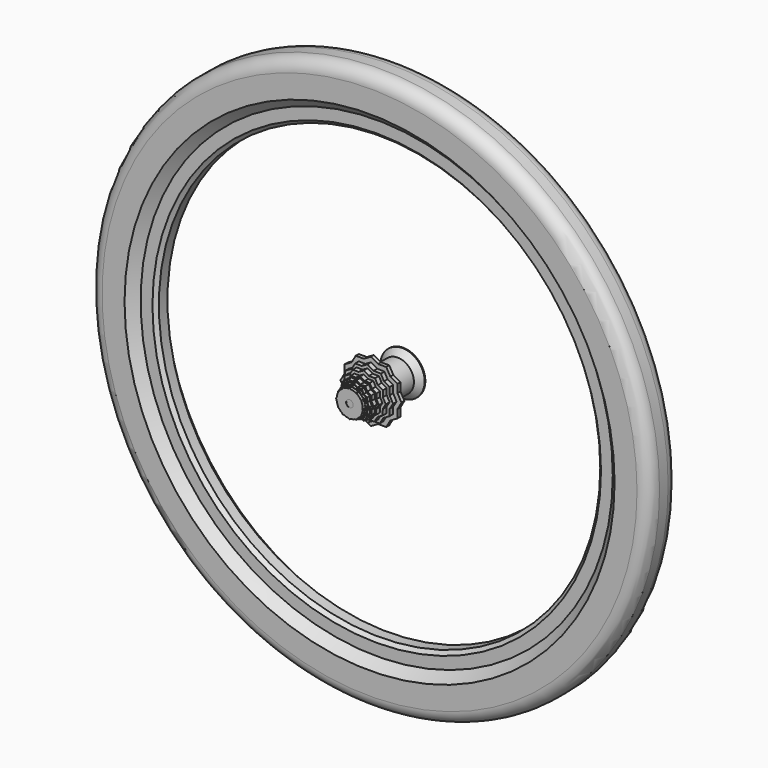
from build123d import *

# Parameters (mm, degrees)
F0_R        = 330.2
F0_R_2      = 313.4398178368
F1_DEPTH    = 12.7
F2_SIZE     = 5.08
F3_R        = 23.0340287743
F4_DEPTH    = 12.7
F5_R        = 31.4850250761
F6_DEPTH    = 21.59
F7_R        = 31.4849467141
F8_DEPTH    = 4.826
F9_S5_R     = 23.0340287743
F9_T6_DEPTH = 47
F10_R       = 18.571291292
F11_DEPTH   = 43.18
F12_R       = 31.4849467141
F13_DEPTH   = 5.334
F15_DEPTH   = 6.35
F17_DEPTH   = 6.858
F19_DEPTH   = 6.35
F21_DEPTH   = 6.35
F23_DEPTH   = 4.572
F25_DEPTH   = 3.302
F27_DEPTH   = 3.8862
F28_R       = 5
F29_DEPTH   = 118.11
F30_R       = 397.6407054021
F30_R_2     = 330.2
F31_DEPTH   = 25.4
F33_R       = 17.78


# Not quite as in the source:
# - a fillet or chamfer that OpenCascade refuses, or shapes differently, is made with other operations: its cross-section is extruded or revolved along the edge and cut away or added


with BuildPart() as f1:
    # F0 (on Front) → F1 (new body, symmetric)
    with BuildSketch(Plane.XZ):
        Circle(F0_R)
        Circle(F0_R_2, mode=Mode.SUBTRACT)
    extrude(amount=F1_DEPTH, both=True)

    # F2
    f2_edges = [f1.edges().sort_by_distance(p)[0] for p in [
        (-313.439818, -12.7, 0),
        (-313.439818, 12.7, 0),
    ]]
    chamfer(f2_edges, length=F2_SIZE)

    # F30 (on Front) → F31 (join, symmetric)
    with BuildSketch(Plane.XZ):
        Circle(F30_R)
        Circle(F30_R_2, mode=Mode.SUBTRACT)
    extrude(amount=F31_DEPTH, both=True)

    # F32: chamfer of 17.78 on 1 edges, made by hand


with BuildPart() as f4:
    # F3 (on Front) → F4 (new body, symmetric)
    with BuildSketch(Plane.XZ):
        Circle(F3_R)
    extrude(amount=F4_DEPTH, both=True)

    # F5 (on face) → F6 (join)
    with BuildSketch(Plane(origin=(0, 12.7, 0), x_dir=(-1, 0, 0), z_dir=(0, 1, 0))):
        Circle(F5_R)
    extrude(amount=F6_DEPTH)

    # F7 (on face) → F8 (join)
    with BuildSketch(Plane.XZ.offset(12.7)):
        Circle(F7_R)
    extrude(amount=F8_DEPTH)

    # F9: chamfer of 20.32 on 1 edges, made by hand


with BuildPart() as f9_tool2:
    # F9_s3 → F9_t4 (revolve)
    with BuildSketch(Plane.XY):
        Polygon((-11.1650250761, 12.7), (-31.4850250761, 33.02), (-31.4850250761, 12.7), align=None)
    revolve(axis=Axis((0, 12.7, 0), (0, 1, 0)))

    # F9_s5 → F9_t6 (cut, symmetric)
    with BuildSketch(Plane.XZ.offset(-22.9)):
        Circle(F9_S5_R)
    extrude(amount=F9_T6_DEPTH, both=True, mode=Mode.SUBTRACT)


with BuildPart() as f4_1:
    add(f4.part)

    # F9_t1: cut F9_tool2
    add(f9_tool2.part, mode=Mode.SUBTRACT)

    # F10 (on face) → F11 (join)
    with BuildSketch(Plane.XZ.offset(17.526)):
        Circle(F10_R)
    extrude(amount=F11_DEPTH)

    # F28 (on face) → F29 (cut)
    with BuildSketch(Plane.XZ.offset(60.706)):
        Circle(F28_R)
    extrude(amount=-F29_DEPTH, mode=Mode.SUBTRACT)


with BuildPart() as f13:
    # F12 (on face) → F13 (new body)
    with BuildSketch(Plane.XZ.offset(17.526)):
        Polygon((37.5246405602, -10.0546971344), (37.5246405602, 10.0546971344), (27.4699434258, 27.4699434258), (10.0546971344, 37.5246405602), (-10.0546971344, 37.5246405602), (-27.4699434258, 27.4699434258), (-37.5246405602, 10.0546971344), (-37.5246405602, -10.0546971344), (-27.4699434258, -27.4699434258), (-10.0546971344, -37.5246405602), (10.0546971344, -37.5246405602), (27.4699434258, -27.4699434258), align=None)
        Circle(F12_R, mode=Mode.SUBTRACT)
        Polygon((10.0546971344, 37.5246405602), (27.4699434258, 27.4699434258), (21.6648613286, 37.5246405602), align=None)
        Polygon((-27.4699434258, 27.4699434258), (-10.0546971344, 37.5246405602), (-21.6648613286, 37.5246405602), align=None)
        Polygon((-10.0546971344, 37.5246405602), (10.0546971344, 37.5246405602), (0, 43.3297226573), align=None)
        Polygon((-37.5246405602, 10.0546971344), (-27.4699434258, 27.4699434258), (-37.5246405602, 21.6648613286), align=None)
        Polygon((-37.5246405602, -10.0546971344), (-37.5246405602, 10.0546971344), (-43.3297226573, 0), align=None)
        Polygon((-37.5246405602, -21.6648613286), (-27.4699434258, -27.4699434258), (-37.5246405602, -10.0546971344), align=None)
        Polygon((-21.6648613286, -37.5246405602), (-10.0546971344, -37.5246405602), (-27.4699434258, -27.4699434258), align=None)
        Polygon((0, -43.3297226573), (10.0546971344, -37.5246405602), (-10.0546971344, -37.5246405602), align=None)
        Polygon((21.6648613286, -37.5246405602), (27.4699434258, -27.4699434258), (10.0546971344, -37.5246405602), align=None)
        Polygon((37.5246405602, -21.6648613286), (37.5246405602, -10.0546971344), (27.4699434258, -27.4699434258), align=None)
        Polygon((43.3297226573, 0), (37.5246405602, 10.0546971344), (37.5246405602, -10.0546971344), align=None)
        Polygon((37.5246405602, 10.0546971344), (37.5246405602, 21.6648613286), (27.4699434258, 27.4699434258), align=None)
    extrude(amount=F13_DEPTH)


with BuildPart() as f15:
    # F14 (on face) → F15 (new body)
    with BuildSketch(Plane.XZ.offset(22.86)):
        Polygon((31.4849467141, 7.9340602855), (31.4849467141, 18.1778424608), (23.487088156, 22.7954082522), align=None)
        Polygon((36.3394488072, -1.0864099174), (31.4849467141, 7.9340602855), (31.4849467141, -8.9427108779), align=None)
        Polygon((31.4849467141, -8.9427108779), (31.4849467141, 7.9340602855), (23.487088156, 22.7954082522), (8.8713755946, 31.2337938339), (-7.9978585581, 31.7381191301), (-22.6135711195, 23.2997335484), (-31.4849467141, 8.9427108779), (-31.4849467141, -7.9340602855), (-23.487088156, -22.7954082522), (-8.8713755946, -31.2337938339), (7.9978585581, -31.7381191301), (22.6135711195, -23.2997335484), align=None)
        Polygon((8.8713755946, 31.2337938339), (23.487088156, 22.7954082522), (19.110582991, 30.9276808678), align=None)
        Polygon((31.4849467141, -18.1778424608), (31.4849467141, -8.9427108779), (22.6135711195, -23.2997335484), align=None)
        Polygon((-7.9978585581, 31.7381191301), (8.8713755946, 31.2337938339), (0, 36.3556849216), align=None)
        Polygon((17.2288658162, -32.0140907852), (22.6135711195, -23.2997335484), (7.9978585581, -31.7381191301), align=None)
        Polygon((-22.6135711195, 23.2997335484), (-7.9978585581, 31.7381191301), (-17.2288658162, 32.0140907852), align=None)
        Polygon((0, -36.3556849216), (7.9978585581, -31.7381191301), (-8.8713755946, -31.2337938339), align=None)
        Polygon((-31.4849467141, 8.9427108779), (-22.6135711195, 23.2997335484), (-31.4849467141, 18.1778424608), align=None)
        Polygon((-19.110582991, -30.9276808678), (-8.8713755946, -31.2337938339), (-23.487088156, -22.7954082522), align=None)
        Polygon((-31.4849467141, -7.9340602855), (-31.4849467141, 8.9427108779), (-36.3394488072, 1.0864099174), align=None)
        Polygon((-31.4849467141, -18.1778424608), (-23.487088156, -22.7954082522), (-31.4849467141, -7.9340602855), align=None)
    extrude(amount=F15_DEPTH)


with BuildPart() as f17:
    # F16 (on face) → F17 (new body)
    with BuildSketch(Plane.XZ.offset(29.21)):
        Polygon((7.6229792377, 27.1815358473), (0.1521180714, 31.5430119156), (-7.0145946523, 27.451262981), align=None)
        Polygon((16.272305085, 27.0221543892), (7.6229792377, 27.1815358473), (20.2661937814, 19.8004486566), align=None)
        Polygon((20.2661937814, 19.8004486566), (7.6229792377, 27.1815358473), (-7.0145946523, 27.451262981), (-19.7284109388, 20.1924615961), (-27.2807884337, 7.6508143244), (-27.3513901765, -6.9890742513), (-20.2661937814, -19.8004486566), (-7.6229792377, -27.1815358473), (7.0145946523, -27.451262981), (19.7284109388, -20.1924615961), (27.2807884337, -7.6508143244), (27.3513901765, 6.9890742513), align=None)
        Polygon((-19.7284109388, 20.1924615961), (-7.0145946523, 27.451262981), (-15.2657196236, 27.6033067763), align=None)
        Polygon((27.3931086665, 15.6397678436), (20.2661937814, 19.8004486566), (27.3513901765, 6.9890742513), align=None)
        Polygon((-27.2807884337, 7.6508143244), (-19.7284109388, 20.1924615961), (-27.2409905951, 15.903244072), align=None)
        Polygon((31.5380247085, -0.5811523871), (27.3513901765, 6.9890742513), (27.2807884337, -7.6508143244), align=None)
        Polygon((-27.3513901765, -6.9890742513), (-27.2807884337, 7.6508143244), (-31.5380247085, 0.5811523871), align=None)
        Polygon((27.2409905951, -15.903244072), (27.2807884337, -7.6508143244), (19.7284109388, -20.1924615961), align=None)
        Polygon((-20.2661937814, -19.8004486566), (-27.3513901765, -6.9890742513), (-27.3931086665, -15.6397678436), align=None)
        Polygon((15.2657196236, -27.6033067763), (19.7284109388, -20.1924615961), (7.0145946523, -27.451262981), align=None)
        Polygon((-7.6229792377, -27.1815358473), (-20.2661937814, -19.8004486566), (-16.272305085, -27.0221543892), align=None)
        Polygon((-0.1521180714, -31.5430119156), (7.0145946523, -27.451262981), (-7.6229792377, -27.1815358473), align=None)
    extrude(amount=F17_DEPTH)


with BuildPart() as f19:
    # F18 (on face) → F19 (new body)
    with BuildSketch(Plane.XZ.offset(36.068)):
        Polygon((6.6182012985, 23.1333943168), (0.4520852324, 26.8332787451), (-5.8351667066, 23.3432078034), align=None)
        Polygon((13.8081566685, 23.0122584439), (6.6182012985, 23.1333943168), (17.2982276102, 16.7250065049), align=None)
        Polygon((17.2982276102, 16.7250065049), (6.6182012985, 23.1333943168), (-5.8351667066, 23.3432078034), (-16.7250065049, 17.2982276102), (-23.1333943168, 6.6182012985), (-23.3432078034, -5.8351667066), (-17.2982276102, -16.7250065049), (-6.6182012985, -23.1333943168), (5.8351667066, -23.3432078034), (16.7250065049, -17.2982276102), (23.1333943168, -6.6182012985), (23.3432078034, 5.8351667066), align=None)
        Polygon((-16.7250065049, 17.2982276102), (-5.8351667066, 23.3432078034), (-13.0251220766, 23.4643436763), align=None)
        Polygon((23.4643436763, 13.0251220766), (17.2982276102, 16.7250065049), (23.3432078034, 5.8351667066), align=None)
        Polygon((-23.1333943168, 6.6182012985), (-16.7250065049, 17.2982276102), (-23.0122584439, 13.8081566685), align=None)
        Polygon((26.8332787451, -0.4520852324), (23.3432078034, 5.8351667066), (23.1333943168, -6.6182012985), align=None)
        Polygon((-23.3432078034, -5.8351667066), (-23.1333943168, 6.6182012985), (-26.8332787451, 0.4520852324), align=None)
        Polygon((23.0122584439, -13.8081566685), (23.1333943168, -6.6182012985), (16.7250065049, -17.2982276102), align=None)
        Polygon((-17.2982276102, -16.7250065049), (-23.3432078034, -5.8351667066), (-23.4643436763, -13.0251220766), align=None)
        Polygon((13.0251220766, -23.4643436763), (16.7250065049, -17.2982276102), (5.8351667066, -23.3432078034), align=None)
        Polygon((-6.6182012985, -23.1333943168), (-17.2982276102, -16.7250065049), (-13.8081566685, -23.0122584439), align=None)
        Polygon((-0.4520852324, -26.8332787451), (5.8351667066, -23.3432078034), (-6.6182012985, -23.1333943168), align=None)
    extrude(amount=F19_DEPTH)


with BuildPart() as f21:
    # F20 (on face) → F21 (new body)
    with BuildSketch(Plane.XZ.offset(42.418)):
        Polygon((15.6329888137, 15.4468506512), (12.497079395, 21.0376595296), (5.795126247, 21.1209169034), align=None)
        Polygon((21.1858358601, 12.2442015171), (15.6329888137, 15.4468506512), (21.1888137131, 5.5417319036), align=None)
        Polygon((21.1888137131, 5.5417319036), (15.6329888137, 15.4468506512), (5.795126247, 21.1209169034), (-5.5608706655, 21.2619907753), (-15.393687466, 15.5791849997), (-21.1938594792, 5.8151401242), (-21.1888137131, -5.5417319036), (-15.6329888137, -15.4468506512), (-5.795126247, -21.1209169034), (5.5608706655, -21.2619907753), (15.393687466, -15.5791849997), (21.1938594792, -5.8151401242), align=None)
        Polygon((-5.5608706655, 21.2619907753), (5.795126247, 21.1209169034), (-0.0108716328, 24.4695728139), align=None)
        Polygon((24.4676872862, -0.3039584644), (21.1888137131, 5.5417319036), (21.1938594792, -5.8151401242), align=None)
        Polygon((-15.393687466, 15.5791849997), (-5.5608706655, 21.2619907753), (-11.9706078913, 21.3416179939), align=None)
        Polygon((21.196707493, -12.2253712967), (21.1938594792, -5.8151401242), (15.393687466, -15.5791849997), align=None)
        Polygon((-21.1938594792, 5.8151401242), (-15.393687466, 15.5791849997), (-21.196707493, 12.2253712967), align=None)
        Polygon((11.9706078913, -21.3416179939), (15.393687466, -15.5791849997), (5.5608706655, -21.2619907753), align=None)
        Polygon((-21.1888137131, -5.5417319036), (-21.1938594792, 5.8151401242), (-24.4676872862, 0.3039584644), align=None)
        Polygon((0.0108716328, -24.4695728139), (5.5608706655, -21.2619907753), (-5.795126247, -21.1209169034), align=None)
        Polygon((-15.6329888137, -15.4468506512), (-21.1888137131, -5.5417319036), (-21.1858358601, -12.2442015171), align=None)
        Polygon((-12.497079395, -21.0376595296), (-5.795126247, -21.1209169034), (-15.6329888137, -15.4468506512), align=None)
    extrude(amount=F21_DEPTH)


with BuildPart() as f23:
    # F22 (on face) → F23 (new body)
    with BuildSketch(Plane.XZ.offset(48.768)):
        Polygon((14.1206154101, 13.8263447779), (11.4125081967, 18.7722549839), (5.2812427209, 18.9111061399), align=None)
        Polygon((19.0084046936, 11.0146925297), (14.1206154101, 13.8263447779), (19.0181196913, 4.8818627101), align=None)
        Polygon((19.0181196913, 4.8818627101), (14.1206154101, 13.8263447779), (5.2812427209, 18.9111061399), (-4.9136581141, 19.1419840512), (-13.7368769704, 14.0292434299), (-19.0342735242, 5.3156392733), (-19.0181196913, -4.8818627101), (-14.1206154101, -13.8263447779), (-5.2812427209, -18.9111061399), (4.9136581141, -19.1419840512), (13.7368769704, -14.0292434299), (19.0342735242, -5.3156392733), align=None)
        Polygon((-4.9136581141, 19.1419840512), (5.2812427209, 18.9111061399), (-0.0348011988, 21.969107615), align=None)
        Polygon((21.9635038007, -0.4973945273), (19.0181196913, 4.8818627101), (19.0342735242, -5.3156392733), align=None)
        Polygon((-13.7368769704, 14.0292434299), (-4.9136581141, 19.1419840512), (-10.550995604, 19.2696495112), align=None)
        Polygon((19.0432058924, -10.9544150852), (19.0342735242, -5.3156392733), (13.7368769704, -14.0292434299), align=None)
        Polygon((-19.0342735242, 5.3156392733), (-13.7368769704, 14.0292434299), (-19.0432058924, 10.9544150852), align=None)
        Polygon((10.550995604, -19.2696495112), (13.7368769704, -14.0292434299), (4.9136581141, -19.1419840512), align=None)
        Polygon((-19.0181196913, -4.8818627101), (-19.0342735242, 5.3156392733), (-21.9635038007, 0.4973945273), align=None)
        Polygon((0.0348011988, -21.969107615), (4.9136581141, -19.1419840512), (-5.2812427209, -18.9111061399), align=None)
        Polygon((-14.1206154101, -13.8263447779), (-19.0181196913, -4.8818627101), (-19.0084046936, -11.0146925297), align=None)
        Polygon((-11.4125081967, -18.7722549839), (-5.2812427209, -18.9111061399), (-14.1206154101, -13.8263447779), align=None)
    extrude(amount=F23_DEPTH)


with BuildPart() as f25:
    # F24 (on face) → F25 (new body)
    with BuildSketch(Plane.XZ.offset(53.34)):
        Polygon((4.9557047364, 17.8605892728), (-0.0098370627, 20.7243044155), (-4.6617860124, 18.0355554854), align=None)
        Polygon((10.686899955, 17.7563244966), (4.9557047364, 17.8605892728), (13.2883562156, 13.0550028564), align=None)
        Polygon((13.2883562156, 13.0550028564), (4.9557047364, 17.8605892728), (-4.6617860124, 18.0355554854), (-12.9898716686, 13.2220608318), (-17.9501422279, 4.980552629), (-17.945576405, -4.638528441), (-13.2883562156, -13.0550028564), (-4.9557047364, -17.8605892728), (4.6617860124, -18.0355554854), (12.9898716686, -13.2220608318), (17.9501422279, -4.980552629), (17.945576405, 4.638528441), align=None)
        Polygon((-12.9898716686, 13.2220608318), (-4.6617860124, 18.0355554854), (-10.0339781144, 18.133289097), align=None)
        Polygon((17.9428555683, 10.370671354), (13.2883562156, 13.0550028564), (17.945576405, 4.638528441), align=None)
        Polygon((-17.9501422279, 4.980552629), (-12.9898716686, 13.2220608318), (-17.952692631, 10.3536330616), align=None)
        Polygon((20.7208780694, -0.3769646005), (17.945576405, 4.638528441), (17.9501422279, -4.980552629), align=None)
        Polygon((-17.945576405, -4.638528441), (-17.9501422279, 4.980552629), (-20.7208780694, 0.3769646005), align=None)
        Polygon((17.952692631, -10.3536330616), (17.9501422279, -4.980552629), (12.9898716686, -13.2220608318), align=None)
        Polygon((-13.2883562156, -13.0550028564), (-17.945576405, -4.638528441), (-17.9428555683, -10.370671354), align=None)
        Polygon((10.0339781144, -18.133289097), (12.9898716686, -13.2220608318), (4.6617860124, -18.0355554854), align=None)
        Polygon((-4.9557047364, -17.8605892728), (-13.2883562156, -13.0550028564), (-10.686899955, -17.7563244966), align=None)
        Polygon((0.0098370627, -20.7243044155), (4.6617860124, -18.0355554854), (-4.9557047364, -17.8605892728), align=None)
    extrude(amount=F25_DEPTH)


with BuildPart() as f27:
    # F26 (on face) → F27 (new body)
    with BuildSketch(Plane.XZ.offset(56.642)):
        Polygon((4.7735277821, 16.8202055695), (0.0513016488, 19.5631203379), (-4.3039365876, 17.0638273834), align=None)
        Polygon((10.2326060501, 16.6736943307), (4.7735277821, 16.8202055695), (12.625739706, 12.2592321128), align=None)
        Polygon((12.625739706, 12.2592321128), (4.7735277821, 16.8202055695), (-4.3039365876, 17.0638273834), (-12.179961429, 12.5440991097), (-16.9296762936, 4.8045952705), (-16.9534892111, -4.2761064598), (-12.625739706, -12.2592321128), (-4.7735277821, -16.8202055695), (4.3039365876, -17.0638273834), (12.179961429, -12.5440991097), (16.9296762936, -4.8045952705), (16.9534892111, 4.2761064598), align=None)
        Polygon((-12.179961429, 12.5440991097), (-4.3039365876, 17.0638273834), (-9.3235398403, 17.1985439517), align=None)
        Polygon((16.9678100143, 9.7371316378), (12.625739706, 12.2592321128), (16.9534892111, 4.2761064598), align=None)
        Polygon((-16.9296762936, 4.8045952705), (-12.179961429, 12.5440991097), (-16.9165083655, 9.8259887001), align=None)
        Polygon((19.5561458904, -0.524849621), (16.9534892111, 4.2761064598), (16.9296762936, -4.8045952705), align=None)
        Polygon((-16.9534892111, -4.2761064598), (-16.9296762936, 4.8045952705), (-19.5561458904, 0.524849621), align=None)
        Polygon((16.9165083655, -9.8259887001), (16.9296762936, -4.8045952705), (12.179961429, -12.5440991097), align=None)
        Polygon((-12.625739706, -12.2592321128), (-16.9534892111, -4.2761064598), (-16.9678100143, -9.7371316378), align=None)
        Polygon((9.3235398403, -17.1985439517), (12.179961429, -12.5440991097), (4.3039365876, -17.0638273834), align=None)
        Polygon((-4.7735277821, -16.8202055695), (-12.625739706, -12.2592321128), (-10.2326060501, -16.6736943307), align=None)
        Polygon((-0.0513016488, -19.5631203379), (4.3039365876, -17.0638273834), (-4.7735277821, -16.8202055695), align=None)
    extrude(amount=F27_DEPTH)


with BuildPart() as f32_tool2:
    # F32_s3 → F32_t4 (revolve)
    with BuildSketch(Plane.XY):
        Polygon((347.98, -25.4), (330.2, -7.62), (330.2, -25.4), align=None)
    revolve(axis=Axis((0, -25.4, 0), (0, -1, 0)))

    split(bisect_by=Plane.XZ.offset(12.7), keep=Keep.TOP)


with BuildPart() as f1_1:
    add(f1.part)

    # F32_t1: cut F32_tool2
    add(f32_tool2.part, mode=Mode.SUBTRACT)

    # F33
    f33_edges = [f1_1.edges().sort_by_distance(p)[0] for p in [
        (-397.640705, -25.4, 0),
        (-397.640705, 25.4, 0),
    ]]
    fillet(f33_edges, radius=F33_R)


solid = Compound([f4_1.part, f13.part, f15.part, f17.part, f19.part, f21.part, f23.part, f25.part, f27.part, f1_1.part])
